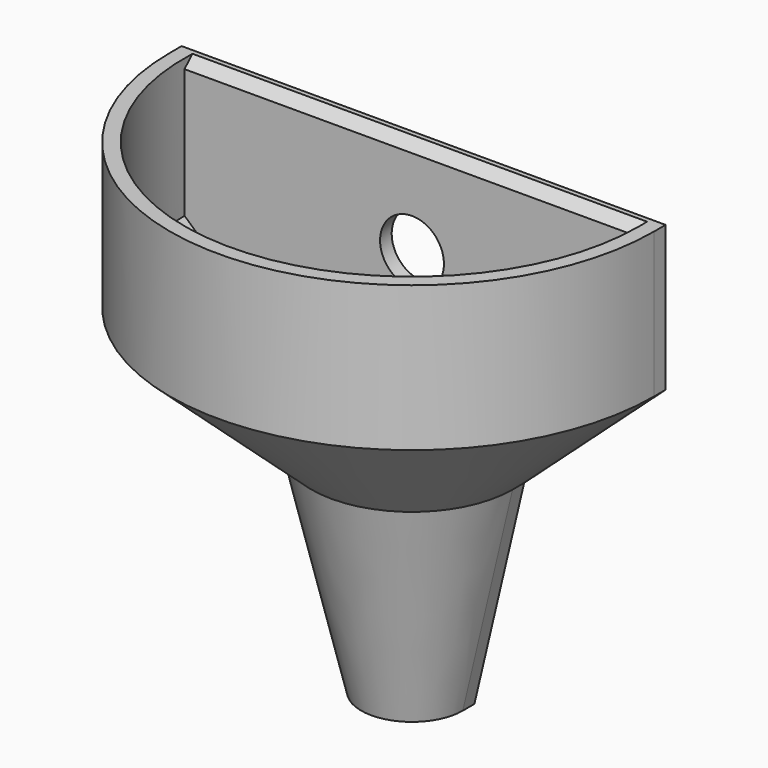
from build123d import *

# Parameters (mm, degrees)
F2_W        = 80.1923088729
F2_H        = 33.5576944053
F3_DEPTH    = 69.4
F5_DEPTH    = 1.5
F6_R        = 3.3
F7_DEPTH    = 3
F8_T4_DEPTH = 52.1433659759
F8_S5_R     = 23.5
F8_T6_DEPTH = 28


# Not quite as in the source:
# - a fillet or chamfer that OpenCascade refuses, or shapes differently, is made with other operations: its cross-section is extruded or revolved along the edge and cut away or added


with BuildPart() as f1:
    # F0 (on Front) → F1 (revolve)
    with BuildSketch(Plane.XZ):
        Polygon((-23.5, 35.6656860253), (-23.5, 48.5), (-23.5, 50), (-25, 50), (-25, 35), (-10.384612577, 21.7765538924), (-5.247530064, 0), (-3.5904949309, 0), (-8.884612577, 22.4422399178), align=None)
    revolve(axis=Axis((0, 0, 32.1634635329), (0, 0, 1)))

    # F2 (on Top) → F3 (cut)
    with BuildSketch(Plane.XY):
        with Locations((8.9423079044, 16.7788472027)):
            Rectangle(F2_W, F2_H)
    extrude(amount=F3_DEPTH, mode=Mode.SUBTRACT)

    # F4 (on face) → F5 (join)
    with BuildSketch(Plane(origin=(0, 0, 0), x_dir=(-1, 0, 0), z_dir=(0, 1, 0))):
        Polygon((25, 50), (-25, 50), (-25, 35), (-10.384612577, 21.7765538924), (-5.247530064, 0), (5.247530064, 0), (10.384612577, 21.7765538924), (25, 35), align=None)
    extrude(amount=F5_DEPTH)

    # F6 (on face) → F7 (cut)
    with BuildSketch(Plane(origin=(0, 1.5, 0), x_dir=(-1, 0, 0), z_dir=(0, 1, 0))):
        with Locations((0, 40)):
            Circle(F6_R)
        with Locations((0, 10)):
            Circle(F6_R)
    extrude(amount=-F7_DEPTH, mode=Mode.SUBTRACT)

    # F8: chamfer of 1 on 1 edges, made by hand


with BuildPart() as f8_tool2:
    # F8_s3 → F8_t4 (new body)
    with BuildSketch(Plane.YZ.offset(-26.071682988)):
        Polygon((0, 49), (1, 50), (0, 50), align=None)
    extrude(amount=F8_T4_DEPTH)

    # F8_s5 → F8_t6 (intersect, symmetric)
    with BuildSketch(Plane.XY.offset(49.5)):
        Circle(F8_S5_R)
    extrude(amount=F8_T6_DEPTH, both=True, mode=Mode.INTERSECT)


with BuildPart() as f1_1:
    add(f1.part)

    # F8_t1: cut F8_tool2
    add(f8_tool2.part, mode=Mode.SUBTRACT)


solid = f1_1.part
